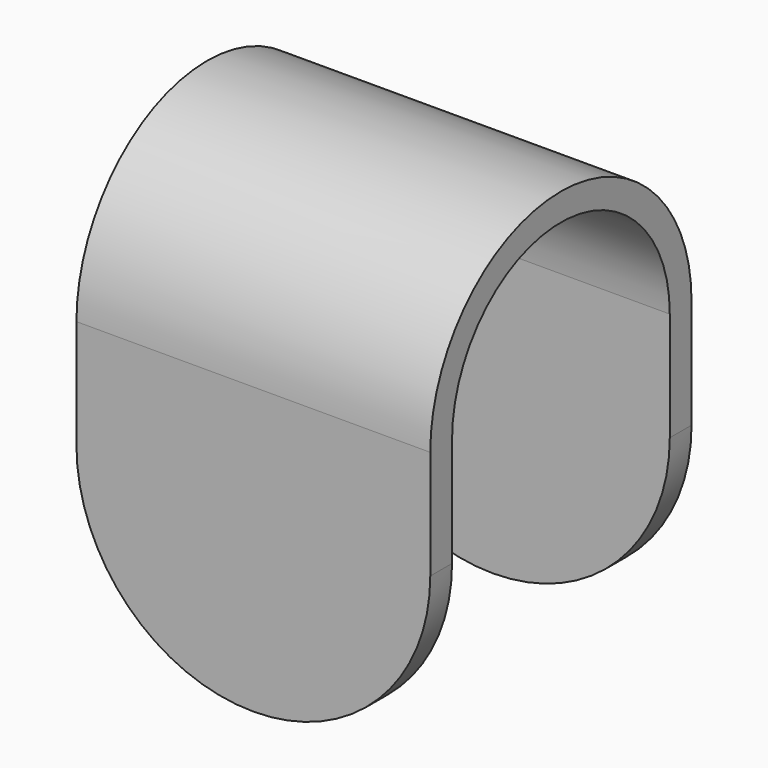
from build123d import *

# Parameters (mm, degrees)
F1_DEPTH = 41.275
F2_R     = 41.27499


# Not quite as in the source:
# - a fillet or chamfer is up to 0.001 mm smaller than in the source, because OpenCascade refuses the exact size


with BuildPart() as f1:
    # F0 (on Right) → F1 (new body, symmetric)
    with BuildSketch(Plane.YZ):
        with BuildLine():
            ThreePointArc((38.1, 0), (0, 38.1), (-38.1, 0))
            Line((-38.1, 0), (-38.1, -66.675))
            Line((-38.1, -66.675), (-31.75, -66.675))
            Line((-31.75, -66.675), (-31.75, 0))
            ThreePointArc((-31.75, 0), (0, 31.75), (31.75, 0))
            Line((31.75, 0), (31.75, -66.675))
            Line((31.75, -66.675), (38.1, -66.675))
            Line((38.1, -66.675), (38.1, 0))
        make_face()
    extrude(amount=F1_DEPTH, both=True)

    # F2 (radius 41.275 in the source; OpenCascade refuses exactly that, so slightly less here)
    f2_edges = [f1.edges().sort_by_distance(p)[0] for p in [
        (-41.275, 34.925, -66.675),
        (-41.275, -34.925, -66.675),
        (41.275, -34.925, -66.675),
        (41.275, 34.925, -66.675),
    ]]
    fillet(f2_edges, radius=F2_R)


solid = f1.part
